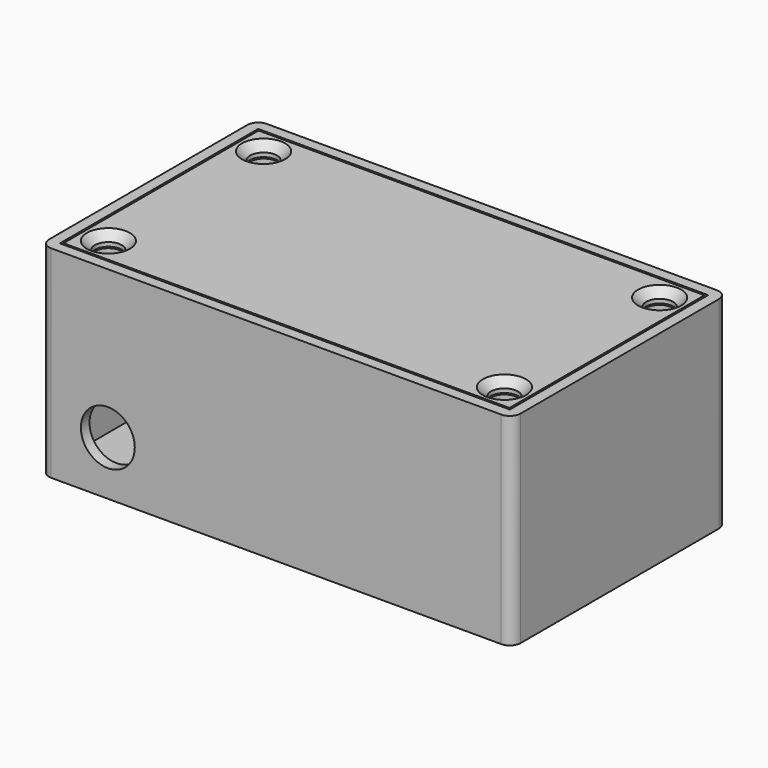
from build123d import *

# Parameters (mm, degrees)
F0_W        = 70
F0_H        = 40
F1_DEPTH    = 30
F2_T        = -1.6
F4_W        = 8
F4_H        = 8
F4_R        = 2
F5_DEPTH    = 10
F6_T1_DEPTH = 28.5734639037
F6_T3_DEPTH = 28.5734639037
F7_R        = 4
F8_DEPTH    = 1.6
F9_W        = 66.2
F9_H        = 36.2
F9_R        = 2
F10_DEPTH   = 1.8
F11_SIZE    = 1.2
F12_R       = 1.6


# Not quite as in the source:
# - a fillet or chamfer that OpenCascade refuses, or shapes differently, is made with other operations: its cross-section is extruded or revolved along the edge and cut away or added


with BuildPart() as f1:
    # F0 (on Top) → F1 (new body)
    with BuildSketch(Plane.XY):
        with Locations((-35, 20)):
            Rectangle(F0_W, F0_H)
    extrude(amount=F1_DEPTH)

    # F2
    f2_openings = [f1.faces().sort_by_distance(p)[0] for p in [
        (-35, 20, 30),
    ]]
    offset(amount=F2_T, openings=f2_openings)

    # F4 (on offset) → F5 (join)
    with BuildSketch(Plane.XY.offset(28)):
        with Locations((-64.4, 34.4)):
            Rectangle(F4_W, F4_H)
        with Locations((-64.4, 34.4)):
            Circle(F4_R, mode=Mode.SUBTRACT)
        with Locations((-5.6, 34.4)):
            Rectangle(F4_W, F4_H)
        with Locations((-5.6, 34.4)):
            Circle(F4_R, mode=Mode.SUBTRACT)
        with Locations((-5.6, 5.6)):
            Rectangle(F4_W, F4_H)
        with Locations((-5.6, 5.6)):
            Circle(F4_R, mode=Mode.SUBTRACT)
        with Locations((-64.4, 5.6)):
            Rectangle(F4_W, F4_H)
        with Locations((-64.4, 5.6)):
            Circle(F4_R, mode=Mode.SUBTRACT)
    extrude(amount=-F5_DEPTH)

    # F6: chamfer of 8 on 4 edges, made by hand

    # F6_s2 → F6_t1 (cut)
    with BuildSketch(Plane.XZ.offset(-38.4)):
        Polygon((-68.4, 18), (-60.4, 26), (-60.4, 18), align=None)
        Polygon((-9.6, 26), (-1.6, 18), (-9.6, 18), align=None)
    extrude(amount=F6_T1_DEPTH, mode=Mode.SUBTRACT)

    # F6_s4 → F6_t3 (cut)
    with BuildSketch(Plane.XZ.offset(-30.1734639037)):
        Polygon((-60.4, 26), (-68.4, 18), (-60.4, 18), align=None)
        Polygon((-1.6, 18), (-9.6, 26), (-9.6, 18), align=None)
    extrude(amount=F6_T3_DEPTH, mode=Mode.SUBTRACT)

    # F7 (on face) → F8 (cut, through all)
    with BuildSketch(Plane.XZ):
        with Locations((-60, 8)):
            Circle(F7_R)
    extrude(amount=-F8_DEPTH, mode=Mode.SUBTRACT)

    # F12
    f12_edges = [f1.edges().sort_by_distance(p)[0] for p in [
        (-70, 0, 15),
        (0, 0, 15),
        (0, 40, 15),
        (-70, 40, 15),
    ]]
    fillet(f12_edges, radius=F12_R)


with BuildPart() as f10:
    # F9 (on face) → F10 (new body)
    with BuildSketch(Plane.XY.offset(30)):
        with Locations((-35, 20)):
            Rectangle(F9_W, F9_H)
        with Locations((-64.4, 5.6)):
            Circle(F9_R, mode=Mode.SUBTRACT)
        with Locations((-5.6, 5.6)):
            Circle(F9_R, mode=Mode.SUBTRACT)
        with Locations((-64.4, 34.4)):
            Circle(F9_R, mode=Mode.SUBTRACT)
        with Locations((-5.6, 34.4)):
            Circle(F9_R, mode=Mode.SUBTRACT)
    extrude(amount=-F10_DEPTH)

    # F11
    f11_edges = [f10.edges().sort_by_distance(p)[0] for p in [
        (-66.4, 34.4, 30),
        (-7.6, 34.4, 30),
        (-7.6, 5.6, 30),
        (-66.4, 5.6, 30),
    ]]
    chamfer(f11_edges, length=F11_SIZE)


solid = Compound([f1.part, f10.part])
